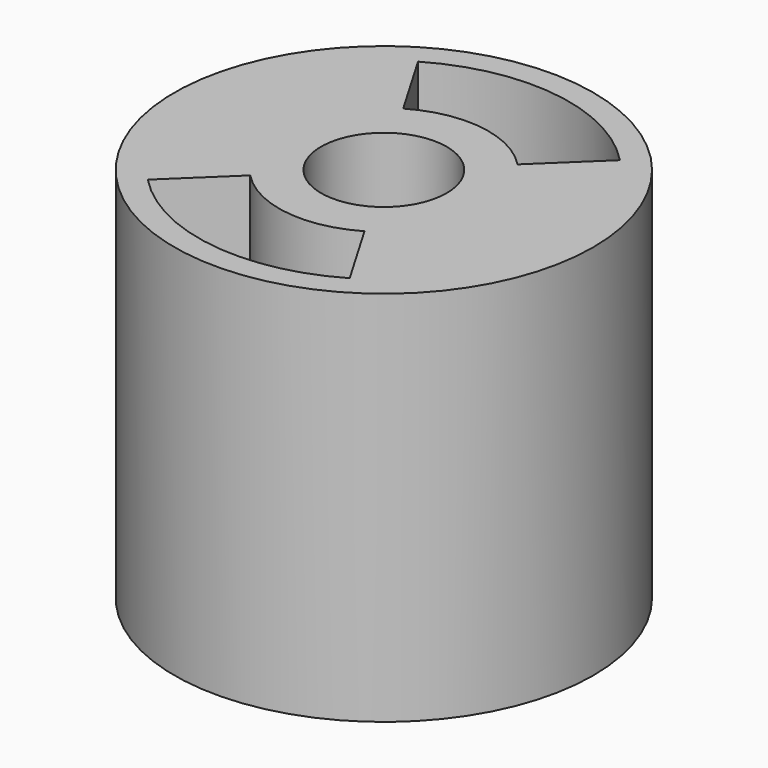
from build123d import *

# Parameters (mm, degrees)
F0_R     = 5
F0_R_2   = 1.5
F1_DEPTH = 9


# Not quite as in the source:
# - a feature names something its author has since deleted; it is built from what else it names


with BuildPart() as f1:
    # F0 (on Top) → F1 (new body)
    with BuildSketch(Plane.XY):
        Circle(F0_R)
        with BuildLine():
            ThreePointArc((-1.8067647919, -1.7300678361), (-0.3453428308, -2.4775536442), (1.2647834859, -2.1582067706))
            Line((1.2647834859, -2.1582067706), (2.2340463063, -3.8121416967))
            ThreePointArc((2.2340463063, -3.8121416967), (-0.6099952159, -4.3762190359), (-3.1913732702, -3.0558998452))
            Line((-3.1913732702, -3.0558998452), (-1.8067647919, -1.7300678361))
        make_face(mode=Mode.SUBTRACT)
        Circle(F0_R_2, mode=Mode.SUBTRACT)
        with BuildLine():
            ThreePointArc((-2.2340463063, 3.8121416967), (0.6099952159, 4.3762190359), (3.1913732702, 3.0558998452))
            Line((3.1913732702, 3.0558998452), (1.8067647919, 1.7300678361))
            ThreePointArc((1.8067647919, 1.7300678361), (0.3453428308, 2.4775536442), (-1.2647834859, 2.1582067706))
            Line((-1.2647834859, 2.1582067706), (-2.2340463063, 3.8121416967))
        make_face(mode=Mode.SUBTRACT)
    extrude(amount=F1_DEPTH)


solid = f1.part
